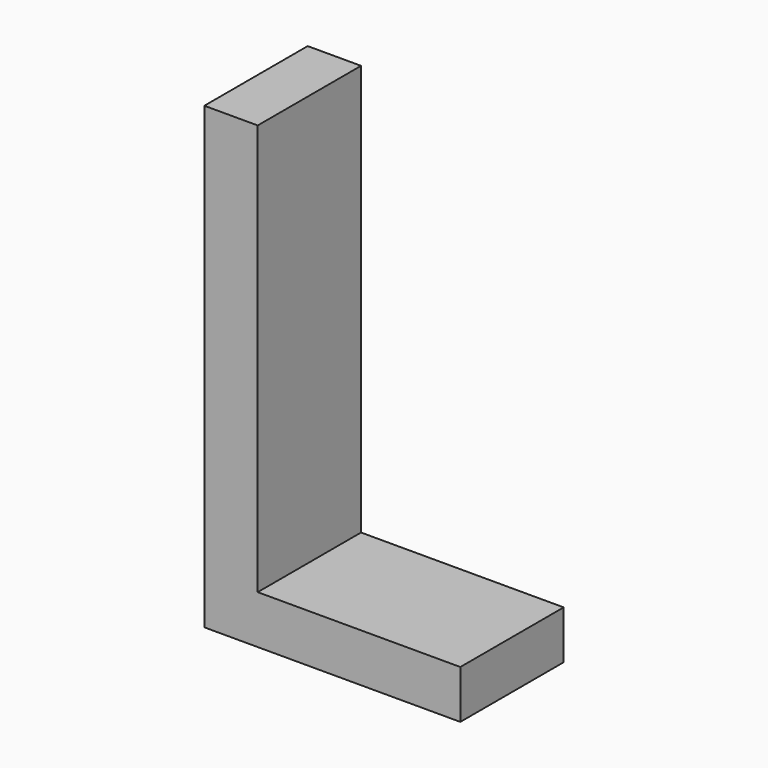
from build123d import *

# Parameters (mm, degrees)
F0_TEXT_SIZE = 124.4882328643
F1_DEPTH     = 25


# Not quite as in the source:
# - Text() gives the source's letters only with a copy of the font that has no kerning and outlines rounded to 1/6400 em; it was checked with that copy


with BuildPart() as f1:
    # F0 (on Front) → F1 (new body)
    with BuildSketch(Plane.XZ):
        with Locations((-54.7300428152, -48.2834093273)):
            Text('L', F0_TEXT_SIZE, font='Open Sans', text_align=(TextAlign.LEFT, TextAlign.BOTTOM))
    extrude(amount=F1_DEPTH)


solid = f1.part
